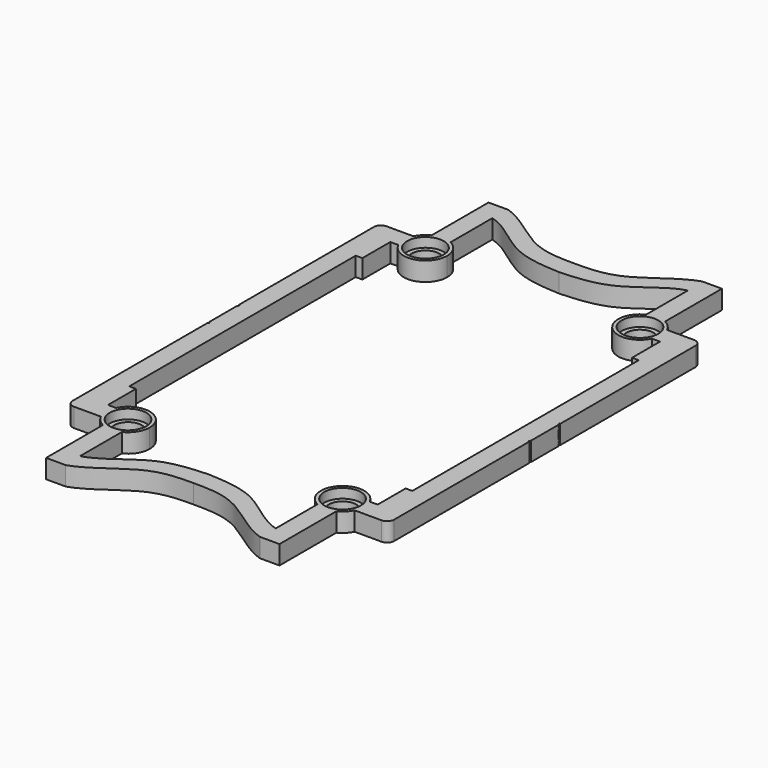
from build123d import *

# Parameters (mm, degrees)
F1_R     = 1.9385702654
F2_DEPTH = 2
F1_R_2   = 1.45
F3_DEPTH = 1


# Not quite as in the source:
# - a feature names something its author has since deleted; it is built from what else it names


with BuildPart() as f2:
    # F1 (on Top) → F2 (new body)
    with BuildSketch(Plane.XY):
        with BuildLine():
            Line((20.1431754695, 54.826795375), (17.2922195872, 54.826795375))
            Line((17.2922195872, 54.826795375), (17.2922195872, 52.826795375))
            Line((17.2922195872, 52.826795375), (19.2922195872, 52.826795375))
            Line((19.2922195872, 52.826795375), (20.1431754695, 52.826795375))
            ThreePointArc((20.1431754695, 52.826795375), (19.9144440108, 53.826795375), (20.1431754695, 54.826795375))
        make_face()
        with BuildLine():
            Line((17.2922195872, 52.826795375), (17.2922195872, 54.826795375))
            ThreePointArc((17.2922195872, 54.826795375), (16.7618895013, 54.6071254609), (16.5422195872, 54.076795375))
            Line((16.5422195872, 54.076795375), (16.5422195872, 36.1640515577))
            Line((16.5422195872, 36.1640515577), (16.6310362357, 36.1640515577))
            add(Edge.make_bspline(
                [(16.6310362357, 36.1640515577), (16.6605582728, 36.102992123), (16.6182720198, 36.0400576616), (16.5422195872, 35.9722101398)],
                knots=[0, 0, 0, 0, 0.1783856354, 0.1783856354, 0.1783856354, 0.1783856354], degree=3))
            Line((16.5422195872, 35.9722101398), (16.5422195872, 34.8729174655))
            add(Edge.make_bspline(
                [(17.2922195872, 35.0191108741), (17.0997972988, 34.9422994833), (16.8549828965, 34.8916378751), (16.5422195872, 34.8729174655)],
                knots=[0.8658058325, 0.8658058325, 0.8658058325, 0.8658058325, 0.9922819661, 0.9922819661, 0.9922819661, 0.9922819661], degree=3))
            Line((17.2922195872, 35.0191108741), (17.2922195872, 38.9486732266))
            Line((17.2922195872, 38.9486732266), (17.2922195872, 52.826795375))
        make_face()
        with BuildLine():
            add(Edge.make_bspline(
                [(23.2901408764, 63.432044637), (25.2347933568, 62.8245805128), (28.7105504794, 59.3608919111), (32.0888348452, 59.3416892775), (33.5841990847, 59.3350770114)],
                knots=[0.341159936, 0.341159936, 0.341159936, 0.341159936, 0.6993169326, 1, 1, 1, 1], degree=3))
            Line((23.2901408764, 63.432044637), (23.214779273, 63.432044637))
            Line((23.214779273, 63.432044637), (23.214779273, 61.432044637))
            add(Edge.make_bspline(
                [(23.214779273, 61.432044637), (25.2803065411, 60.8475667943), (28.1242407781, 57.3282649057), (33.0082662404, 57.3930760622), (33.5841990847, 57.3350770114)],
                knots=[0, 0, 0, 0, 0.5448236167, 1, 1, 1, 1], degree=3))
            Line((33.5841990847, 57.3350770114), (33.5841990847, 59.3350770114))
        make_face()
        with BuildLine():
            Line((19.2922195872, 52.826795375), (17.2922195872, 52.826795375))
            Line((17.2922195872, 52.826795375), (17.2922195872, 38.9486732266))
            add(Edge.make_bspline(
                [(17.2922195872, 38.9486732266), (17.9578883588, 37.6855991358), (18.2133900062, 36.1544678124), (17.7506952192, 35.2021258003), (17.2922195872, 35.0191108741)],
                knots=[0, 0, 0, 0, 0.5644570346, 0.8658058325, 0.8658058325, 0.8658058325, 0.8658058325], degree=3))
            Line((17.2922195872, 35.0191108741), (17.2922195872, 34.1235491752))
            Line((17.2922195872, 34.1235491752), (18.5841990847, 34.1235491752))
            Line((18.5841990847, 34.1235491752), (18.5841990847, 49.1235491752))
            Line((18.5841990847, 49.1235491752), (19.2922195872, 49.1235491752))
            Line((19.2922195872, 49.1235491752), (19.2922195872, 52.826795375))
        make_face()
        with BuildLine():
            ThreePointArc((21.214779273, 55.8983991785), (20.5881966101, 55.4533780379), (20.1431754695, 54.826795375))
            ThreePointArc((20.1431754695, 54.826795375), (19.9144440108, 53.826795375), (20.1431754695, 52.826795375))
            ThreePointArc((20.1431754695, 52.826795375), (22.7276920531, 51.5843719542), (24.5151145351, 53.826795375))
            ThreePointArc((24.5151145351, 53.826795375), (24.1630961851, 55.0497440772), (23.214779273, 55.8983991785))
            ThreePointArc((23.214779273, 55.8983991785), (22.214779273, 56.1271306372), (21.214779273, 55.8983991785))
        make_face()
        with Locations((22.214779273, 53.826795375)):
            Circle(F1_R, mode=Mode.SUBTRACT)
        with BuildLine():
            Line((23.214779273, 63.432044637), (21.214779273, 63.432044637))
            Line((21.214779273, 63.432044637), (21.214779273, 55.8983991785))
            ThreePointArc((21.214779273, 55.8983991785), (22.214779273, 56.1271306372), (23.214779273, 55.8983991785))
            Line((23.214779273, 55.8983991785), (23.214779273, 61.432044637))
            Line((23.214779273, 61.432044637), (23.214779273, 63.432044637))
        make_face()
        with BuildLine():
            add(Edge.make_bspline(
                [(43.8782572929, 63.432044637), (41.9336048125, 62.8245805128), (38.4578476899, 59.3608919111), (35.0795633241, 59.3416892775), (33.5841990847, 59.3350770114)],
                knots=[0.341159936, 0.341159936, 0.341159936, 0.341159936, 0.6993169326, 1, 1, 1, 1], degree=3))
            Line((33.5841990847, 59.3350770114), (33.5841990847, 57.3350770114))
            add(Edge.make_bspline(
                [(43.9536188964, 61.432044637), (41.8880916283, 60.8475667943), (39.0441573912, 57.3282649057), (34.160131929, 57.3930760622), (33.5841990847, 57.3350770114)],
                knots=[0, 0, 0, 0, 0.5448236167, 1, 1, 1, 1], degree=3))
            Line((43.9536188964, 61.432044637), (43.9536188964, 63.432044637))
            Line((43.9536188964, 63.432044637), (43.8782572929, 63.432044637))
        make_face()
        with BuildLine():
            add(Edge.make_bspline(
                [(17.2922195872, 38.9486732266), (17.9578883588, 37.6855991358), (18.2133900062, 36.1544678124), (17.7506952192, 35.2021258003), (17.2922195872, 35.0191108741)],
                knots=[0, 0, 0, 0, 0.5644570346, 0.8658058325, 0.8658058325, 0.8658058325, 0.8658058325], degree=3))
            Line((17.2922195872, 38.9486732266), (17.2922195872, 35.0191108741))
        make_face()
        with BuildLine():
            Line((17.2922195872, 34.1235491752), (17.2922195872, 35.0191108741))
            add(Edge.make_bspline(
                [(17.2922195872, 35.0191108741), (17.0997972988, 34.9422994833), (16.8549828965, 34.8916378751), (16.5422195872, 34.8729174655)],
                knots=[0.8658058325, 0.8658058325, 0.8658058325, 0.8658058325, 0.9922819661, 0.9922819661, 0.9922819661, 0.9922819661], degree=3))
            Line((16.5422195872, 34.8729174655), (16.5422195872, 34.1235491752))
            Line((16.5422195872, 34.1235491752), (17.2922195872, 34.1235491752))
        make_face()
        with BuildLine():
            Line((45.9536188964, 63.432044637), (43.9536188964, 63.432044637))
            Line((43.9536188964, 63.432044637), (43.9536188964, 61.432044637))
            Line((43.9536188964, 61.432044637), (43.9536188964, 55.8983991785))
            ThreePointArc((43.9536188964, 55.8983991785), (44.9536188964, 56.1271306372), (45.9536188964, 55.8983991785))
            Line((45.9536188964, 55.8983991785), (45.9536188964, 63.432044637))
        make_face()
        with BuildLine():
            Line((17.2922195872, 33.2279874763), (17.2922195872, 34.1235491752))
            Line((17.2922195872, 34.1235491752), (16.5422195872, 34.1235491752))
            Line((16.5422195872, 34.1235491752), (16.5422195872, 33.3741808849))
            add(Edge.make_bspline(
                [(17.2922195872, 33.2279874763), (17.0997972989, 33.304798867), (16.8549828965, 33.3554604753), (16.5422195872, 33.3741808849)],
                knots=[0.8658058325, 0.8658058325, 0.8658058325, 0.8658058325, 0.9922819661, 0.9922819661, 0.9922819661, 0.9922819661], degree=3))
        make_face()
        with BuildLine():
            Line((18.5841990847, 34.1235491752), (17.2922195872, 34.1235491752))
            Line((17.2922195872, 34.1235491752), (17.2922195872, 33.2279874763))
            add(Edge.make_bspline(
                [(17.2922195872, 29.2984251514), (17.9578883575, 30.5614992398), (18.213390004, 32.092630538), (17.7506952207, 33.0449725495), (17.2922195872, 33.2279874763)],
                knots=[0, 0, 0, 0, 0.5644570335, 0.8658058325, 0.8658058325, 0.8658058325, 0.8658058325], degree=3))
            Line((17.2922195872, 29.2984251514), (17.2922195872, 15.4203029754))
            Line((17.2922195872, 15.4203029754), (19.2922195872, 15.4203029754))
            Line((19.2922195872, 15.4203029754), (19.2922195872, 19.1235491752))
            Line((19.2922195872, 19.1235491752), (18.5841990847, 19.1235491752))
            Line((18.5841990847, 19.1235491752), (18.5841990847, 34.1235491752))
        make_face()
        with BuildLine():
            Line((47.8761785822, 52.826795375), (47.8761785822, 49.1235491752))
            Line((47.8761785822, 49.1235491752), (48.5841990847, 49.1235491752))
            Line((48.5841990847, 49.1235491752), (48.5841990847, 34.1235491752))
            Line((48.5841990847, 34.1235491752), (49.8755873878, 34.1235491752))
            Line((49.8755873878, 34.1235491752), (49.8755873878, 35.0193505084))
            add(Edge.make_bspline(
                [(49.8755873878, 38.9486732266), (49.2099248299, 37.685610926), (48.955176546, 36.1546772336), (49.4175949717, 35.2024133246), (49.8755873878, 35.0193505084)],
                knots=[0, 0, 0, 0, 0.5644517657, 0.8656719041, 0.8656719041, 0.8656719041, 0.8656719041], degree=3))
            Line((49.8755873878, 38.9486732266), (49.8755873878, 52.826795375))
            Line((49.8755873878, 52.826795375), (47.8761785822, 52.826795375))
        make_face()
        with BuildLine():
            ThreePointArc((45.9536188964, 55.8983991785), (44.9536188964, 56.1271306372), (43.9536188964, 55.8983991785))
            ThreePointArc((43.9536188964, 55.8983991785), (43.3270362335, 52.2002127122), (47.0252226998, 52.826795375))
            ThreePointArc((47.0252226998, 52.826795375), (47.1960423172, 53.3138825949), (47.2539541585, 53.826795375))
            ThreePointArc((47.2539541585, 53.826795375), (47.1960423172, 54.3397081552), (47.0252226998, 54.826795375))
            ThreePointArc((47.0252226998, 54.826795375), (46.5802015593, 55.4533780379), (45.9536188964, 55.8983991785))
        make_face()
        with Locations((44.9536188964, 53.826795375)):
            Circle(F1_R, mode=Mode.SUBTRACT)
        with BuildLine():
            Line((17.2922195872, 29.2984251514), (17.2922195872, 33.2279874763))
            add(Edge.make_bspline(
                [(17.2922195872, 33.2279874763), (17.0997972989, 33.304798867), (16.8549828965, 33.3554604753), (16.5422195872, 33.3741808849)],
                knots=[0.8658058325, 0.8658058325, 0.8658058325, 0.8658058325, 0.9922819661, 0.9922819661, 0.9922819661, 0.9922819661], degree=3))
            Line((16.5422195872, 33.3741808849), (16.5422195872, 32.2748882106))
            add(Edge.make_bspline(
                [(16.6310362357, 32.0830467928), (16.6605582728, 32.1441062274), (16.6182720198, 32.2070406889), (16.5422195872, 32.2748882106)],
                knots=[0, 0, 0, 0, 0.1783856354, 0.1783856354, 0.1783856354, 0.1783856354], degree=3))
            Line((16.6310362357, 32.0830467928), (16.5422195872, 32.0830467928))
            Line((16.5422195872, 32.0830467928), (16.5422195872, 14.1703029754))
            ThreePointArc((16.5422195872, 14.1703029754), (16.7618895013, 13.6399728895), (17.2922195872, 13.4203029754))
            Line((17.2922195872, 13.4203029754), (17.2922195872, 14.4203029754))
            Line((17.2922195872, 14.4203029754), (17.2922195872, 15.4203029754))
            Line((17.2922195872, 15.4203029754), (17.2922195872, 29.2984251514))
        make_face()
        with BuildLine():
            add(Edge.make_bspline(
                [(17.2922195872, 29.2984251514), (17.9578883575, 30.5614992398), (18.213390004, 32.092630538), (17.7506952207, 33.0449725495), (17.2922195872, 33.2279874763)],
                knots=[0, 0, 0, 0, 0.5644570335, 0.8658058325, 0.8658058325, 0.8658058325, 0.8658058325], degree=3))
            Line((17.2922195872, 33.2279874763), (17.2922195872, 29.2984251514))
        make_face()
        with BuildLine():
            Line((49.8755873878, 34.1235491752), (48.5841990847, 34.1235491752))
            Line((48.5841990847, 34.1235491752), (48.5841990847, 19.1235491752))
            Line((48.5841990847, 19.1235491752), (47.8761785822, 19.1235491752))
            Line((47.8761785822, 19.1235491752), (47.8761785822, 15.4203029754))
            Line((47.8761785822, 15.4203029754), (49.8755873878, 15.4203029754))
            Line((49.8755873878, 15.4203029754), (49.8755873878, 29.2984251238))
            add(Edge.make_bspline(
                [(49.8755873878, 29.2984251238), (49.2099248299, 30.5614874244), (48.955176546, 32.0924211168), (49.4175949717, 33.0446850258), (49.8755873878, 33.227747842)],
                knots=[0, 0, 0, 0, 0.5644517657, 0.8656719041, 0.8656719041, 0.8656719041, 0.8656719041], degree=3))
            Line((49.8755873878, 33.227747842), (49.8755873878, 34.1235491752))
        make_face()
        with BuildLine():
            Line((47.0252226998, 52.826795375), (47.8761785822, 52.826795375))
            Line((47.8761785822, 52.826795375), (49.8755873878, 52.826795375))
            Line((49.8755873878, 52.826795375), (49.8755873878, 54.826795375))
            Line((49.8755873878, 54.826795375), (47.0252226998, 54.826795375))
            ThreePointArc((47.0252226998, 54.826795375), (47.1960423172, 54.3397081552), (47.2539541585, 53.826795375))
            ThreePointArc((47.2539541585, 53.826795375), (47.1960423172, 53.3138825949), (47.0252226998, 52.826795375))
        make_face()
        with BuildLine():
            Line((49.8761785822, 54.826795375), (49.8755873878, 54.826795375))
            Line((49.8755873878, 54.826795375), (49.8755873878, 52.826795375))
            Line((49.8755873878, 52.826795375), (49.8755873878, 38.9486732266))
            Line((49.8755873878, 38.9486732266), (49.8755873878, 35.0193505084))
            add(Edge.make_bspline(
                [(49.8755873878, 35.0193505084), (50.068092586, 34.9424048157), (50.3130851315, 34.891657493), (50.6261785822, 34.8729174529)],
                knots=[0.8656719041, 0.8656719041, 0.8656719041, 0.8656719041, 0.9922819536, 0.9922819536, 0.9922819536, 0.9922819536], degree=3))
            Line((50.6261785822, 34.8729174529), (50.6261785822, 35.9722101398))
            add(Edge.make_bspline(
                [(50.5373619336, 36.1640515577), (50.5078398965, 36.102992123), (50.5501261495, 36.0400576616), (50.6261785822, 35.9722101398)],
                knots=[0, 0, 0, 0, 0.1783856354, 0.1783856354, 0.1783856354, 0.1783856354], degree=3))
            Line((50.5373619336, 36.1640515577), (50.6261785822, 36.1640515577))
            Line((50.6261785822, 36.1640515577), (50.6261785822, 54.076795375))
            ThreePointArc((50.6261785822, 54.076795375), (50.406508668, 54.6071254609), (49.8761785822, 54.826795375))
        make_face()
        with BuildLine():
            add(Edge.make_bspline(
                [(42.8341990846, 7.271012371), (41.2830937007, 8.0839085723), (38.5430987116, 10.9121843818), (34.160131929, 10.8540222882), (33.5841990847, 10.912021339)],
                knots=[0.1025913324, 0.1025913324, 0.1025913324, 0.1025913324, 0.5448236167, 1, 1, 1, 1], degree=3))
            Line((33.5841990847, 10.912021339), (33.5841990847, 8.912021339))
            add(Edge.make_bspline(
                [(43.8782572929, 4.8150537134), (41.9336048125, 5.4225178376), (38.4578476899, 8.8862064393), (35.0795633241, 8.9054090729), (33.5841990847, 8.912021339)],
                knots=[0.341159936, 0.341159936, 0.341159936, 0.341159936, 0.6993169326, 1, 1, 1, 1], degree=3))
            Line((43.8782572929, 4.8150537134), (43.9536188964, 4.8150537134))
            Line((43.9536188964, 4.8150537134), (43.9536188964, 6.8150537134))
            add(Edge.make_bspline(
                [(43.9536188964, 6.8150537134), (43.5646761486, 6.9251120127), (43.1940325333, 7.0824325062), (42.8341990846, 7.271012371)],
                knots=[0, 0, 0, 0, 0.1025913324, 0.1025913324, 0.1025913324, 0.1025913324], degree=3))
        make_face()
        with BuildLine():
            Line((33.5841990847, 8.912021339), (33.5841990847, 10.912021339))
            add(Edge.make_bspline(
                [(24.3341990847, 7.271012371), (25.8853044686, 8.0839085723), (28.6252994577, 10.9121843818), (33.0082662404, 10.8540222882), (33.5841990847, 10.912021339)],
                knots=[0.1025913324, 0.1025913324, 0.1025913324, 0.1025913324, 0.5448236167, 1, 1, 1, 1], degree=3))
            add(Edge.make_bspline(
                [(23.214779273, 6.8150537134), (23.6037220207, 6.9251120127), (23.974365636, 7.0824325062), (24.3341990847, 7.271012371)],
                knots=[0, 0, 0, 0, 0.1025913324, 0.1025913324, 0.1025913324, 0.1025913324], degree=3))
            Line((23.214779273, 6.8150537134), (23.214779273, 4.8150537134))
            Line((23.214779273, 4.8150537134), (23.2901408764, 4.8150537134))
            add(Edge.make_bspline(
                [(23.2901408764, 4.8150537134), (25.2347933568, 5.4225178376), (28.7105504794, 8.8862064393), (32.0888348452, 8.9054090729), (33.5841990847, 8.912021339)],
                knots=[0.341159936, 0.341159936, 0.341159936, 0.341159936, 0.6993169326, 1, 1, 1, 1], degree=3))
        make_face()
        with BuildLine():
            Line((49.8755873878, 35.0193505084), (49.8755873878, 34.1235491752))
            Line((49.8755873878, 34.1235491752), (50.6261785822, 34.1235491752))
            Line((50.6261785822, 34.1235491752), (50.6261785822, 34.8729174529))
            add(Edge.make_bspline(
                [(49.8755873878, 35.0193505084), (50.068092586, 34.9424048157), (50.3130851315, 34.891657493), (50.6261785822, 34.8729174529)],
                knots=[0.8656719041, 0.8656719041, 0.8656719041, 0.8656719041, 0.9922819536, 0.9922819536, 0.9922819536, 0.9922819536], degree=3))
        make_face()
        with BuildLine():
            Line((50.6261785822, 34.1235491752), (49.8755873878, 34.1235491752))
            Line((49.8755873878, 34.1235491752), (49.8755873878, 33.227747842))
            add(Edge.make_bspline(
                [(49.8755873878, 33.227747842), (50.068092586, 33.3046935347), (50.3130851315, 33.3554408575), (50.6261785822, 33.3741808975)],
                knots=[0.8656719041, 0.8656719041, 0.8656719041, 0.8656719041, 0.9922819536, 0.9922819536, 0.9922819536, 0.9922819536], degree=3))
            Line((50.6261785822, 33.3741808975), (50.6261785822, 34.1235491752))
        make_face()
        with BuildLine():
            Line((19.2922195872, 15.4203029754), (17.2922195872, 15.4203029754))
            Line((17.2922195872, 15.4203029754), (17.2922195872, 14.4203029754))
            Line((17.2922195872, 14.4203029754), (19.9144440108, 14.4203029754))
            ThreePointArc((19.9144440108, 14.4203029754), (19.9723558521, 14.9332157555), (20.1431754695, 15.4203029754))
            Line((20.1431754695, 15.4203029754), (19.2922195872, 15.4203029754))
        make_face()
        with BuildLine():
            Line((49.8755873878, 15.4203029754), (47.8761785822, 15.4203029754))
            Line((47.8761785822, 15.4203029754), (47.0252226998, 15.4203029754))
            ThreePointArc((47.0252226998, 15.4203029754), (47.1960423172, 14.9332157555), (47.2539541585, 14.4203029754))
            ThreePointArc((47.2539541585, 14.4203029754), (47.1960423172, 13.9073901952), (47.0252226998, 13.4203029754))
            Line((47.0252226998, 13.4203029754), (49.8755873878, 13.4203029754))
            Line((49.8755873878, 13.4203029754), (49.8755873878, 15.4203029754))
        make_face()
        with BuildLine():
            add(Edge.make_bspline(
                [(49.8755873878, 38.9486732266), (49.2099248299, 37.685610926), (48.955176546, 36.1546772336), (49.4175949717, 35.2024133246), (49.8755873878, 35.0193505084)],
                knots=[0, 0, 0, 0, 0.5644517657, 0.8656719041, 0.8656719041, 0.8656719041, 0.8656719041], degree=3))
            Line((49.8755873878, 35.0193505084), (49.8755873878, 38.9486732266))
        make_face()
        with BuildLine():
            Line((49.8755873878, 29.2984251238), (49.8755873878, 33.227747842))
            add(Edge.make_bspline(
                [(49.8755873878, 29.2984251238), (49.2099248299, 30.5614874244), (48.955176546, 32.0924211168), (49.4175949717, 33.0446850258), (49.8755873878, 33.227747842)],
                knots=[0, 0, 0, 0, 0.5644517657, 0.8656719041, 0.8656719041, 0.8656719041, 0.8656719041], degree=3))
        make_face()
        with BuildLine():
            add(Edge.make_bspline(
                [(49.8755873878, 33.227747842), (50.068092586, 33.3046935347), (50.3130851315, 33.3554408575), (50.6261785822, 33.3741808975)],
                knots=[0.8656719041, 0.8656719041, 0.8656719041, 0.8656719041, 0.9922819536, 0.9922819536, 0.9922819536, 0.9922819536], degree=3))
            Line((49.8755873878, 33.227747842), (49.8755873878, 29.2984251238))
            Line((49.8755873878, 29.2984251238), (49.8755873878, 15.4203029754))
            Line((49.8755873878, 15.4203029754), (49.8755873878, 13.4203029754))
            Line((49.8755873878, 13.4203029754), (49.8761785822, 13.4203029754))
            ThreePointArc((49.8761785822, 13.4203029754), (50.406508668, 13.6399728895), (50.6261785822, 14.1703029754))
            Line((50.6261785822, 14.1703029754), (50.6261785822, 32.0830467928))
            Line((50.6261785822, 32.0830467928), (50.5373619336, 32.0830467928))
            add(Edge.make_bspline(
                [(50.5373619336, 32.0830467928), (50.5078398965, 32.1441062274), (50.5501261495, 32.2070406889), (50.6261785822, 32.2748882106)],
                knots=[0, 0, 0, 0, 0.1783856354, 0.1783856354, 0.1783856354, 0.1783856354], degree=3))
            Line((50.6261785822, 32.2748882106), (50.6261785822, 33.3741808975))
        make_face()
        with BuildLine():
            Line((19.9144440108, 14.4203029754), (17.2922195872, 14.4203029754))
            Line((17.2922195872, 14.4203029754), (17.2922195872, 13.4203029754))
            Line((17.2922195872, 13.4203029754), (20.1431754695, 13.4203029754))
            ThreePointArc((20.1431754695, 13.4203029754), (19.9723558521, 13.9073901952), (19.9144440108, 14.4203029754))
        make_face()
        with BuildLine():
            Line((43.9536188964, 12.3486991719), (43.9536188964, 6.8150537134))
            Line((43.9536188964, 6.8150537134), (43.9536188964, 4.8150537134))
            Line((43.9536188964, 4.8150537134), (45.9536188964, 4.8150537134))
            Line((45.9536188964, 4.8150537134), (45.9536188964, 12.3486991719))
            ThreePointArc((45.9536188964, 12.3486991719), (44.9536188964, 12.1199677132), (43.9536188964, 12.3486991719))
        make_face()
        with BuildLine():
            Line((23.214779273, 4.8150537134), (23.214779273, 6.8150537134))
            Line((23.214779273, 6.8150537134), (23.214779273, 12.3486991719))
            ThreePointArc((23.214779273, 12.3486991719), (22.7276920531, 12.1778795545), (22.214779273, 12.1199677132))
            Line((22.214779273, 12.1199677132), (22.214779273, 4.8150537134))
            Line((22.214779273, 4.8150537134), (23.214779273, 4.8150537134))
        make_face()
        with BuildLine():
            ThreePointArc((24.5151145351, 14.4203029754), (22.7276920531, 16.6627263962), (20.1431754695, 15.4203029754))
            ThreePointArc((20.1431754695, 15.4203029754), (19.9723558521, 14.9332157555), (19.9144440108, 14.4203029754))
            ThreePointArc((19.9144440108, 14.4203029754), (19.9723558521, 13.9073901952), (20.1431754695, 13.4203029754))
            ThreePointArc((20.1431754695, 13.4203029754), (20.5881966101, 12.7937203125), (21.214779273, 12.3486991719))
            ThreePointArc((21.214779273, 12.3486991719), (21.7018664928, 12.1778795545), (22.214779273, 12.1199677132))
            ThreePointArc((22.214779273, 12.1199677132), (22.7276920531, 12.1778795545), (23.214779273, 12.3486991719))
            ThreePointArc((23.214779273, 12.3486991719), (24.1630961851, 13.1973542732), (24.5151145351, 14.4203029754))
        make_face()
        with Locations((22.214779273, 14.4203029754)):
            Circle(F1_R, mode=Mode.SUBTRACT)
        with BuildLine():
            ThreePointArc((47.2539541585, 14.4203029754), (47.1960423172, 14.9332157555), (47.0252226998, 15.4203029754))
            ThreePointArc((47.0252226998, 15.4203029754), (43.3270362335, 16.0468856383), (43.9536188964, 12.3486991719))
            ThreePointArc((43.9536188964, 12.3486991719), (44.9536188964, 12.1199677132), (45.9536188964, 12.3486991719))
            ThreePointArc((45.9536188964, 12.3486991719), (46.5802015593, 12.7937203125), (47.0252226998, 13.4203029754))
            ThreePointArc((47.0252226998, 13.4203029754), (47.1960423172, 13.9073901952), (47.2539541585, 14.4203029754))
        make_face()
        with Locations((44.9536188964, 14.4203029754)):
            Circle(F1_R, mode=Mode.SUBTRACT)
        with BuildLine():
            Line((21.214779273, 4.8150537134), (22.214779273, 4.8150537134))
            Line((22.214779273, 4.8150537134), (22.214779273, 12.1199677132))
            ThreePointArc((22.214779273, 12.1199677132), (21.7018664928, 12.1778795545), (21.214779273, 12.3486991719))
            Line((21.214779273, 12.3486991719), (21.214779273, 4.8150537134))
        make_face()
    extrude(amount=F2_DEPTH)

    # F1 (on Top) → F3 (join)
    with BuildSketch(Plane.XY):
        with BuildLine():
            ThreePointArc((21.214779273, 55.8983991785), (20.5881966101, 55.4533780379), (20.1431754695, 54.826795375))
            ThreePointArc((20.1431754695, 54.826795375), (19.9144440108, 53.826795375), (20.1431754695, 52.826795375))
            ThreePointArc((20.1431754695, 52.826795375), (22.7276920531, 51.5843719542), (24.5151145351, 53.826795375))
            ThreePointArc((24.5151145351, 53.826795375), (24.1630961851, 55.0497440772), (23.214779273, 55.8983991785))
            ThreePointArc((23.214779273, 55.8983991785), (22.214779273, 56.1271306372), (21.214779273, 55.8983991785))
        make_face()
        with Locations((22.214779273, 53.826795375)):
            Circle(F1_R, mode=Mode.SUBTRACT)
        with BuildLine():
            Line((17.2922195872, 33.2279874763), (17.2922195872, 34.1235491752))
            Line((17.2922195872, 34.1235491752), (16.5422195872, 34.1235491752))
            Line((16.5422195872, 34.1235491752), (16.5422195872, 33.3741808849))
            add(Edge.make_bspline(
                [(17.2922195872, 33.2279874763), (17.0997972989, 33.304798867), (16.8549828965, 33.3554604753), (16.5422195872, 33.3741808849)],
                knots=[0.8658058325, 0.8658058325, 0.8658058325, 0.8658058325, 0.9922819661, 0.9922819661, 0.9922819661, 0.9922819661], degree=3))
        make_face()
        with BuildLine():
            ThreePointArc((47.2539541585, 14.4203029754), (47.1960423172, 14.9332157555), (47.0252226998, 15.4203029754))
            ThreePointArc((47.0252226998, 15.4203029754), (43.3270362335, 16.0468856383), (43.9536188964, 12.3486991719))
            ThreePointArc((43.9536188964, 12.3486991719), (44.9536188964, 12.1199677132), (45.9536188964, 12.3486991719))
            ThreePointArc((45.9536188964, 12.3486991719), (46.5802015593, 12.7937203125), (47.0252226998, 13.4203029754))
            ThreePointArc((47.0252226998, 13.4203029754), (47.1960423172, 13.9073901952), (47.2539541585, 14.4203029754))
        make_face()
        with Locations((44.9536188964, 14.4203029754)):
            Circle(F1_R, mode=Mode.SUBTRACT)
        with Locations((22.214779273, 14.4203029754)):
            Circle(F1_R)
        with Locations((22.214779273, 14.4203029754)):
            Circle(F1_R_2, mode=Mode.SUBTRACT)
        with Locations((22.214779273, 53.826795375)):
            Circle(F1_R)
        with Locations((22.214779273, 53.826795375)):
            Circle(F1_R_2, mode=Mode.SUBTRACT)
        with Locations((44.9536188964, 14.4203029754)):
            Circle(F1_R)
        with Locations((44.9536188964, 14.4203029754)):
            Circle(F1_R_2, mode=Mode.SUBTRACT)
        with Locations((44.9536188964, 53.826795375)):
            Circle(F1_R)
        with Locations((44.9536188964, 53.826795375)):
            Circle(F1_R_2, mode=Mode.SUBTRACT)
    extrude(amount=F3_DEPTH)


solid = f2.part
